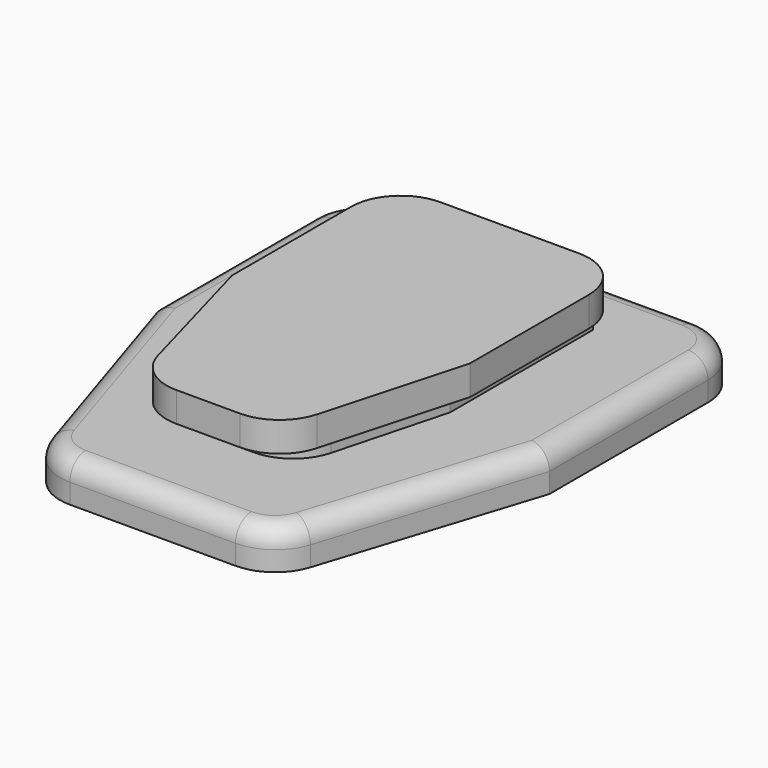
from build123d import *

# Parameters (mm, degrees)
F1_DEPTH        = 4
F2_R            = 5
F3_R            = 2
F5_DEPTH        = 6
F6_R            = 5
F8_DEPTH        = 3
F10_F1_R        = 5
F10_F2_R        = 5
F10_2_T1_DEPTH  = 11.6034789136
F10_2_T3_DEPTH  = 16.5
F10_2_T5_DEPTH  = 13.1244047484
F10_2_T8_ANGLE  = 72.2553283749
F10_2_T10_ANGLE = 90


# Not quite as in the source:
# - a fillet or chamfer that OpenCascade refuses, or shapes differently, is made with other operations: its cross-section is extruded or revolved along the edge and cut away or added
# - a pattern or mirror of a feature is missing from the dataset's text; its kind, count and spacing are read off the source's solid


with BuildPart() as f1:
    # F0 (on Top) → F1 (new body)
    with BuildSketch(Plane.XY):
        Polygon((0, 25), (0, 0), (0, -25), (12, -25), (20, 0), (20, 25), align=None)
    extrude(amount=F1_DEPTH)

    # F1_copies: F1 across plane


with BuildPart() as f1_1:
    add(f1.part)
    add(f1.part.mirror(Plane(origin=(0, 0, 0), x_dir=(0, 0, -1), z_dir=(-1, 0, 0))))

    # F2
    f2_edges = [f1_1.edges().sort_by_distance(p)[0] for p in [
        (12, -25, 2),
        (20, 25, 2),
    ]]
    fillet(f2_edges, radius=F2_R)

    # F3
    f3_edges = [f1_1.edges().sort_by_distance(p)[0] for p in [
        (-1.824881, -25, 4),
        (20, 10, 4),
        (11.29817, -24.038527, 4),
        (-16, -12.5, 4),
        (16.556179, -10.761939, 4),
        (-20, 12.5, 4),
        (-2.5, 25, 4),
        (18.535534, 23.535534, 4),
    ]]
    fillet(f3_edges, radius=F3_R)

    # F4 (on Top) → F5 (join)
    with BuildSketch(Plane.XY):
        Polygon((0, 18), (0, 0), (0, -15), (6, -15), (10, 0), (10, 18), align=None)
    f5 = extrude(amount=F5_DEPTH)

    # F5_copies: F5 across plane
    add(f5.mirror(Plane(origin=(0, 0, 0), x_dir=(0, 0, -1), z_dir=(-1, 0, 0))))

    # F6
    f6_edges = [f1_1.edges().sort_by_distance(p)[0] for p in [
        (6, -15, 5),
    ]]
    fillet(f6_edges, radius=F6_R)

    # F10#2: fillet of radius 5 on 3 edges, made by hand

    # F10_2_s2 → F10_2_t1 (cut)
    with BuildSketch(Plane.XY.offset(4)):
        with BuildLine():
            ThreePointArc((-2.1586084346, -15), (-5.2047891364, -13.9649442785), (-6.9897831326, -11.2883132528))
            Line((-6.9897831326, -11.2883132528), (-6, -15))
            Line((-6, -15), (-2.1586084346, -15))
        make_face()
    extrude(amount=F10_2_T1_DEPTH, mode=Mode.SUBTRACT)

    # F10_2_s4 → F10_2_t3 (cut)
    with BuildSketch(Plane.XY.offset(-12.5)):
        with BuildLine():
            ThreePointArc((-15, 25), (-18.5355339059, 23.5355339059), (-20, 20))
            Line((-20, 20), (-20, 25))
            Line((-20, 25), (-15, 25))
        make_face()
    extrude(amount=F10_2_T3_DEPTH, mode=Mode.SUBTRACT)

    # F10_2_s6 → F10_2_t5 (cut)
    with BuildSketch(Plane.XY.offset(-9.1244047484)):
        with BuildLine():
            ThreePointArc((-13.1123588366, -21.5238786355), (-11.2981701574, -24.0385265368), (-8.3502381006, -25))
            Line((-8.3502381006, -25), (-12, -25))
            Line((-12, -25), (-13.1123588366, -21.5238786355))
        make_face()
    extrude(amount=F10_2_T5_DEPTH, mode=Mode.SUBTRACT)

    # F10_2_s7 → F10_2_t8 (revolve, cut)
    with BuildSketch(Plane(origin=(5.0298762867, -15.718363396, 0), x_dir=(0, 0, 1), z_dir=(-0.3047757271, 0.9524241472, 0))):
        with BuildLine():
            ThreePointArc((4, -17.048482944), (3.4142135624, -18.4626965064), (2, -19.048482944))
            Line((2, -19.048482944), (4, -19.048482944))
            Line((4, -19.048482944), (4, -17.048482944))
        make_face()
    revolve(axis=Axis((-8.3502381006, -20, 4), (0, 0, 1)), revolution_arc=F10_2_T8_ANGLE, mode=Mode.SUBTRACT)

    # F10_2_s9 → F10_2_t10 (revolve, cut)
    with BuildSketch(Plane.YZ.offset(-15)):
        with BuildLine():
            ThreePointArc((23, 4), (24.4142135624, 3.4142135624), (25, 2))
            Line((25, 2), (25, 4))
            Line((25, 4), (23, 4))
        make_face()
    revolve(axis=Axis((-15, 20, 4), (0, 0, 1)), revolution_arc=F10_2_T10_ANGLE, mode=Mode.SUBTRACT)



with BuildPart() as f8:
    # F7 (on Top) → F8 (new body)
    with BuildSketch(Plane.XY):
        Polygon((0, 20), (0, 0), (0, -18), (7, -18), (12, 0), (12, 20), align=None)
    extrude(amount=F8_DEPTH)


with BuildPart() as f8_1:
    # F9: moved
    add(f8.part.moved(Location((0, 0, 6))))

    # F10: fillet of radius 5 on 2 edges, made by hand

    # F10_f1
    f10_f1_edges = [f8_1.edges().sort_by_distance(p)[0] for p in [
        (12, 20, 7.5),
    ]]
    fillet(f10_f1_edges, radius=F10_F1_R)

    # F10_f2
    f10_f2_edges = [f8_1.edges().sort_by_distance(p)[0] for p in [
        (7, -18, 7.5),
    ]]
    fillet(f10_f2_edges, radius=F10_F2_R)


with BuildPart() as f1_2:
    add(f1_1.part)

    add(f8_1.part)  # F11 merges F8
    # F11: F8 across plane
    add(f8_1.part.mirror(Plane.YZ))


solid = f1_2.part
